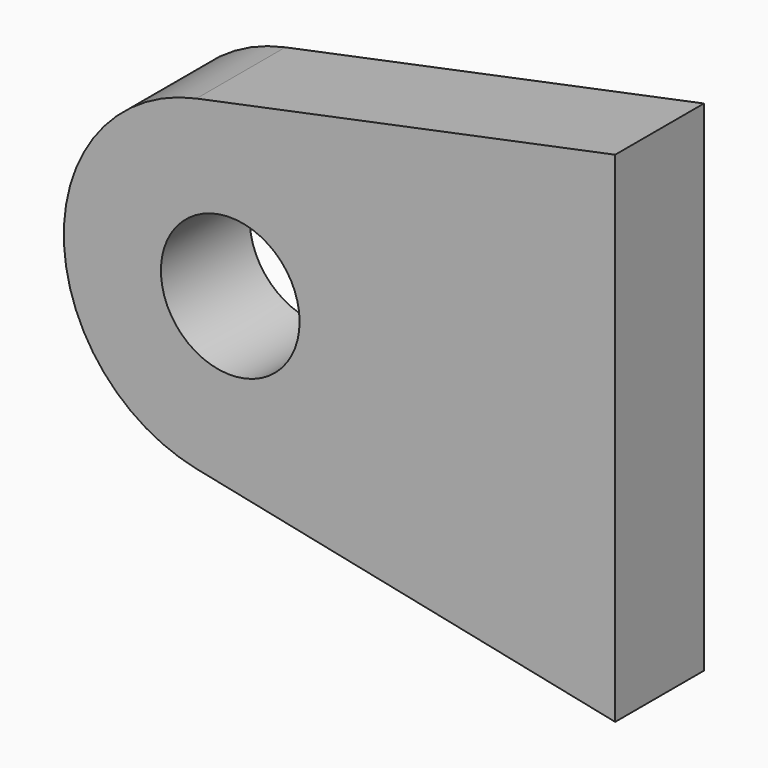
from build123d import *

# Parameters (mm, degrees)
F1_DEPTH = 20
F0_R     = 12.5
F2_DEPTH = 20


# Not quite as in the source:
# - a feature names something its author has since deleted; it is built from what else it names


with BuildPart() as f1:
    # F0 (on Front) → F1 (new body)
    with BuildSketch(Plane.XZ):
        with BuildLine():
            Line((-0.6229226271, -45), (-0.6229226271, 45))
            Line((-0.6229226271, 45), (-76.0821841814, 29.3769813899))
            ThreePointArc((-76.0821841814, 29.3769813899), (-51.0588480477, 23.2644097866), (-40, 0))
            ThreePointArc((-40, 0), (-51.0588480477, -23.2644097866), (-76.0821841814, -29.3769813899))
            Line((-76.0821841814, -29.3769813899), (-0.6229226271, -45))
        make_face()
    extrude(amount=F1_DEPTH)

    # F0 (on Front) → F2 (join)
    with BuildSketch(Plane.XZ):
        with BuildLine():
            ThreePointArc((-40, 0), (-51.0588480477, 23.2644097866), (-76.0821841814, 29.3769813899))
            ThreePointArc((-76.0821841814, 29.3769813899), (-100, 0), (-76.0821841814, -29.3769813899))
            ThreePointArc((-76.0821841814, -29.3769813899), (-51.0588480477, -23.2644097866), (-40, 0))
        make_face()
        with Locations((-70, 0)):
            Circle(F0_R, mode=Mode.SUBTRACT)
    extrude(amount=F2_DEPTH)


solid = f1.part
